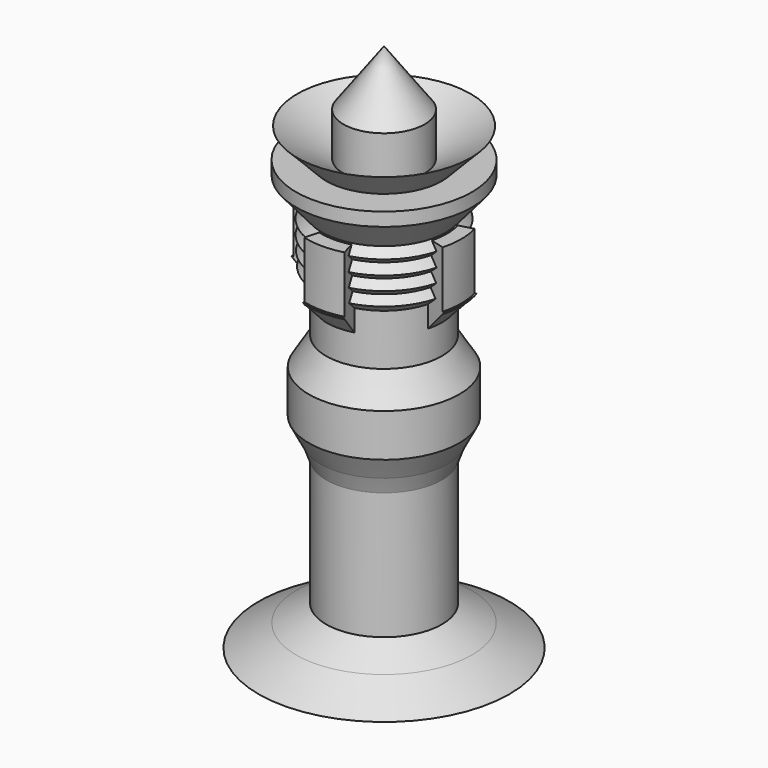
from build123d import *

# Parameters (mm, degrees)
F1_W            = 3.9823013358
F1_H            = 8.4623899311
F3_ANGLE_BACK   = 15
F3_ANGLE        = 30
F3_COPIES_COUNT = 4
F5_ANGLE_BACK   = 15
F5_ANGLE        = 30
F5_COPIES_COUNT = 4


# Not quite as in the source:
# - a pattern or mirror of a feature is missing from the dataset's text; its kind, count and spacing are read off the source's solid


with BuildPart() as f2:
    # F0 (on Front) → F2 (revolve)
    with BuildSketch(Plane.XZ):
        Polygon((0, 57.2826008411), (0, -18.7173991589), (18, -18.7173991589), (12.58260943, -15.5477793887), (8.3016352728, -13.0588412285), (8.3016352728, -4.7955662012), (8.3016352728, 1.6756732948), (8.3016352728, 5.1601859741), (9.1348709539, 7.4490089901), (10.7923932374, 10.6456615031), (10.7923932374, 16.8021768332), (8.3016352728, 20.8275895566), (8.3016352728, 28.1680505723), (9.7421156242, 29.4479895383), (8.7946596922, 30.5142838619), (9.8650568815, 31.4653853958), (8.8950488368, 32.5570605196), (9.914630721, 33.4630101088), (8.9067585183, 34.5972986517), (9.9263404025, 35.5032482409), (8.9067585183, 36.6507151981), (12.6114161685, 41.0112217069), (12.6114161685, 42.9367274046), (8.3016352728, 42.9367274046), (12.4439811334, 47.2063235939), (5.8302935213, 43.1041605771), (5.8302935213, 49.299262464), align=None)
    revolve(axis=Axis((0, 0, 19.2826008411), (0, 0, -1)))

    # F1 (on Front) → F3 (revolve)
    with BuildSketch(Plane.XZ, mode=Mode.PRIVATE) as f3_sk:
        with Locations((9.1009729076, 32.2875799611)):
            Rectangle(F1_W, F1_H)
    f3 = revolve(f3_sk.sketch.rotate(Axis((0, 0, 30.8512914926), (0, 0, -1)), -F3_ANGLE_BACK), axis=Axis((0, 0, 30.8512914926), (0, 0, -1)), revolution_arc=F3_ANGLE)

    # F3_copies: F3 ×4 about axis
    f3_copies_axis = Axis((0, 0, 0), (0, 0, 1))
    for i in range(1, F3_COPIES_COUNT):
        add(f3.rotate(f3_copies_axis, i * 360 / F3_COPIES_COUNT))

    # F4 (on Front) → F5 (revolve)
    with BuildSketch(Plane.XZ, mode=Mode.PRIVATE) as f5_sk:
        Polygon((8.193298243, 24.9484814703), (11.3307544962, 28.381921351), (8.193298243, 28.5003166646), align=None)
    f5 = revolve(f5_sk.sketch.rotate(Axis((0, 0, 30.8512914926), (0, 0, -1)), -F5_ANGLE_BACK), axis=Axis((0, 0, 30.8512914926), (0, 0, -1)), revolution_arc=F5_ANGLE)

    # F5_copies: F5 ×4 about axis
    f5_copies_axis = Axis((0, 0, 0), (0, 0, 1))
    for i in range(1, F5_COPIES_COUNT):
        add(f5.rotate(f5_copies_axis, i * 360 / F5_COPIES_COUNT))


solid = f2.part
